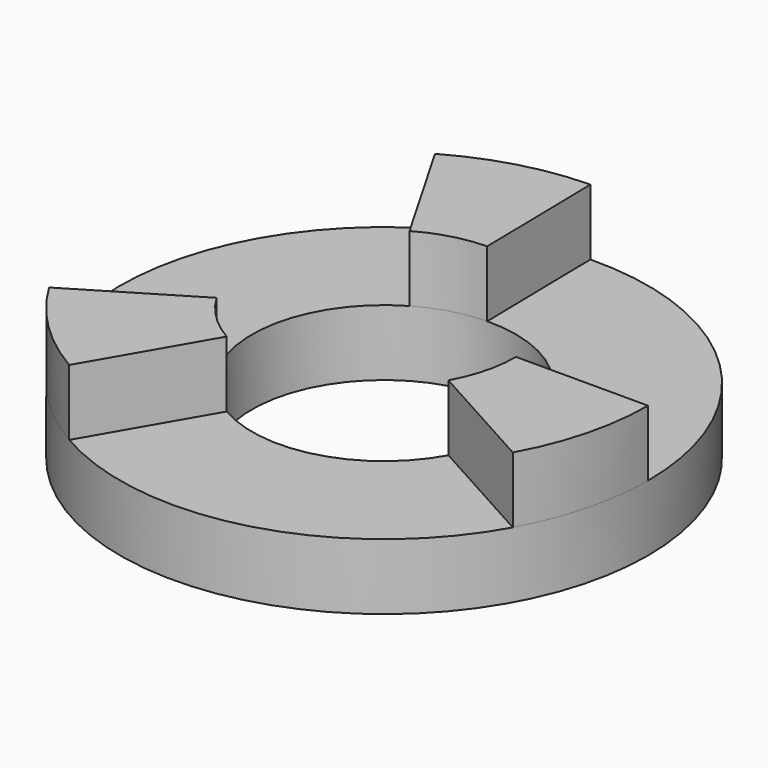
from build123d import *
from build123d import SkipClean  # not in build123d's __all__

# Parameters (mm, degrees)
F0_R     = 20
F0_R_2   = 10
F1_DEPTH = 5
F3_DEPTH = 5


with BuildPart() as f1:
    # F0 (on Top) → F1 (new body)
    with BuildSketch(Plane.XY):
        Circle(F0_R)
        Circle(F0_R_2, mode=Mode.SUBTRACT)
    extrude(amount=F1_DEPTH)

    # F2 (on face) → F3 (join)
    with BuildSketch(Plane.XY.offset(5)):
        with BuildLine():
            ThreePointArc((-5, -8.6602540378), (-7.0062926922, -7.1352549156), (-8.5676274578, -5.1571076917))
            Line((-8.5676274578, -5.1571076917), (-17.1352549156, -10.3142153835))
            ThreePointArc((-17.1352549156, -10.3142153835), (-14.0125853844, -14.2705098312), (-10, -17.3205080757))
            Line((-10, -17.3205080757), (-5, -8.6602540378))
        make_face()
        with BuildLine():
            ThreePointArc((10, 0), (9.6824583655, -2.5), (8.75, -4.8412291828))
            Line((8.75, -4.8412291828), (17.5, -9.6824583655))
            ThreePointArc((17.5, -9.6824583655), (19.364916731, -5), (20, 0))
            Line((20, 0), (10, 0))
        make_face()
        with BuildLine():
            ThreePointArc((-5, 8.6602540378), (-2.6761656733, 9.6352549156), (-0.1823725422, 9.9983368745))
            Line((-0.1823725422, 9.9983368745), (-0.3647450844, 19.996673749))
            ThreePointArc((-0.3647450844, 19.996673749), (-5.3523313466, 19.2705098312), (-10, 17.3205080757))
            Line((-10, 17.3205080757), (-5, 8.6602540378))
        make_face()
    with SkipClean():  # cleaning this boolean's faces spoils the solid; the shape is the same uncleaned
        extrude(amount=F3_DEPTH)


solid = f1.part
